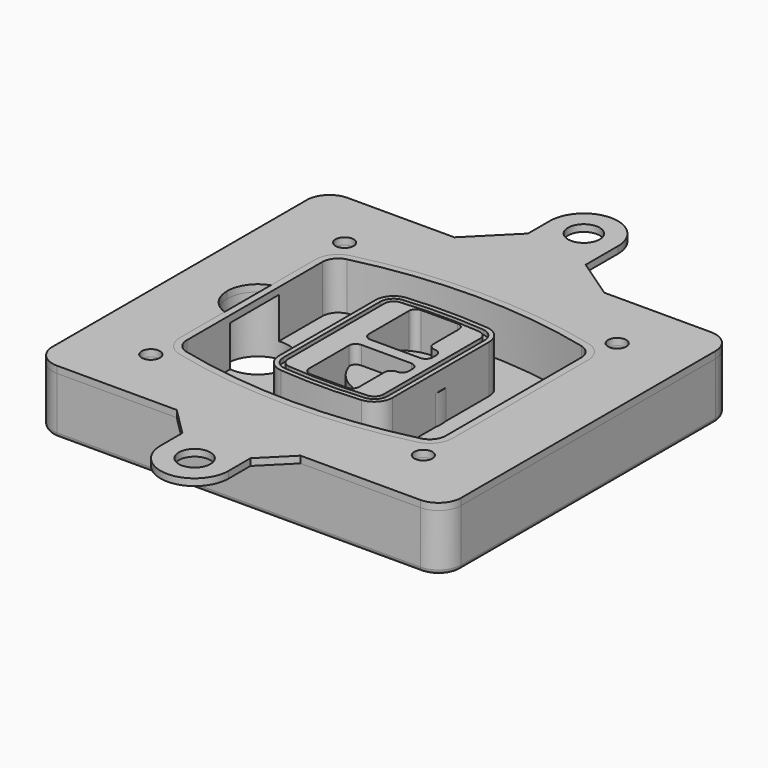
from build123d import *

# Parameters (mm, degrees)
F0_R      = 4
F1_DEPTH  = 25
F2_DEPTH  = 3
F3_DEPTH  = 18
F5_DEPTH  = 21
F6_DEPTH  = 2
F8_DEPTH  = 20
F9_DEPTH  = 16
F10_DEPTH = 25
F7_R      = 6
F7_R_2    = 4
F11_DEPTH = 6
F13_DEPTH = 9
F15_R     = 2
F16_R     = 6.9644805488
F16_R_2   = 4
F17_DEPTH = 3


# Not quite as in the source:
# - a feature of the source that left no trace in its solid (it failed there, or was rolled back) is left out
# - a feature names something its author has since deleted; it is built from what else it names


with BuildPart() as f1:
    # F0 (on Top) → F1 (new body)
    with BuildSketch(Plane.XY):
        with BuildLine():
            ThreePointArc((-90, -70), (-87.0710678119, -77.0710678119), (-80, -80))
            Line((-80, -80), (80, -80))
            ThreePointArc((80, -80), (87.0710678119, -77.0710678119), (90, -70))
            Line((90, -70), (90, 70))
            ThreePointArc((90, 70), (87.0710678119, 77.0710678119), (80, 80))
            Line((80, 80), (-80, 80))
            ThreePointArc((-80, 80), (-87.0710678119, 77.0710678119), (-90, 70))
            Line((-90, 70), (-90, -70))
        make_face()
        with Locations((-60, -53.3333333333)):
            Circle(F0_R, mode=Mode.SUBTRACT)
        with Locations((60, -53.3333333333)):
            Circle(F0_R, mode=Mode.SUBTRACT)
        with Locations((-60, 53.3333333333)):
            Circle(F0_R, mode=Mode.SUBTRACT)
        with BuildLine():
            ThreePointArc((-64, 37.2990447398), (-61.0143011354, 45.9411029726), (-53.3306899286, 50.8970778549))
            ThreePointArc((-53.3306899286, 50.8970778549), (0, 57.3333333333), (53.3306899286, 50.8970778549))
            ThreePointArc((53.3306899286, 50.8970778549), (61.0143011354, 45.9411029726), (64, 37.2990447398))
            Line((64, 37.2990447398), (64, -37.2990447398))
            ThreePointArc((64, -37.2990447398), (61.0143011354, -45.9411029726), (53.3306899286, -50.8970778549))
            ThreePointArc((53.3306899286, -50.8970778549), (0, -57.3333333333), (-53.3306899286, -50.8970778549))
            ThreePointArc((-53.3306899286, -50.8970778549), (-61.0143011354, -45.9411029726), (-64, -37.2990447398))
            Line((-64, -37.2990447398), (-64, 37.2990447398))
        make_face(mode=Mode.SUBTRACT)
        with Locations((60, 53.3333333333)):
            Circle(F0_R, mode=Mode.SUBTRACT)
        with BuildLine():
            ThreePointArc((53.3306899286, 50.8970778549), (0, 57.3333333333), (-53.3306899286, 50.8970778549))
            ThreePointArc((-53.3306899286, 50.8970778549), (-61.0143011354, 45.9411029726), (-64, 37.2990447398))
            Line((-64, 37.2990447398), (-64, -37.2990447398))
            ThreePointArc((-64, -37.2990447398), (-61.0143011354, -45.9411029726), (-53.3306899286, -50.8970778549))
            ThreePointArc((-53.3306899286, -50.8970778549), (0, -57.3333333333), (53.3306899286, -50.8970778549))
            ThreePointArc((53.3306899286, -50.8970778549), (61.0143011354, -45.9411029726), (64, -37.2990447398))
            Line((64, -37.2990447398), (64, 37.2990447398))
            ThreePointArc((64, 37.2990447398), (61.0143011354, 45.9411029726), (53.3306899286, 50.8970778549))
        make_face()
        with BuildLine():
            Line((-60, -37.2990447398), (-60, 37.2990447398))
            ThreePointArc((-60, 37.2990447398), (-57.8673579538, 43.4719434775), (-52.3790642347, 47.0119255363))
            ThreePointArc((-52.3790642347, 47.0119255363), (0, 53.3333333333), (52.3790642347, 47.0119255363))
            ThreePointArc((52.3790642347, 47.0119255363), (57.8673579538, 43.4719434775), (60, 37.2990447398))
            Line((60, 37.2990447398), (60, -37.2990447398))
            ThreePointArc((60, -37.2990447398), (57.8673579538, -43.4719434775), (52.3790642347, -47.0119255363))
            ThreePointArc((52.3790642347, -47.0119255363), (0, -53.3333333333), (-52.3790642347, -47.0119255363))
            ThreePointArc((-52.3790642347, -47.0119255363), (-57.8673579538, -43.4719434775), (-60, -37.2990447398))
        make_face(mode=Mode.SUBTRACT)
        with BuildLine():
            ThreePointArc((-52.3790642347, 47.0119255363), (-57.8673579538, 43.4719434775), (-60, 37.2990447398))
            Line((-60, 37.2990447398), (-60, -37.2990447398))
            ThreePointArc((-60, -37.2990447398), (-57.8673579538, -43.4719434775), (-52.3790642347, -47.0119255363))
            ThreePointArc((-52.3790642347, -47.0119255363), (0, -53.3333333333), (52.3790642347, -47.0119255363))
            ThreePointArc((52.3790642347, -47.0119255363), (57.8673579538, -43.4719434775), (60, -37.2990447398))
            Line((60, -37.2990447398), (60, 37.2990447398))
            ThreePointArc((60, 37.2990447398), (57.8673579538, 43.4719434775), (52.3790642347, 47.0119255363))
            ThreePointArc((52.3790642347, 47.0119255363), (0, 53.3333333333), (-52.3790642347, 47.0119255363))
        make_face()
        with BuildLine():
            ThreePointArc((51.6653449643, 44.0980612973), (55.5071505677, 41.6200738562), (57, 37.2990447398))
            Line((57, 37.2990447398), (57, -37.2990447398))
            ThreePointArc((57, -37.2990447398), (55.5071505677, -41.6200738562), (51.6653449643, -44.0980612973))
            ThreePointArc((51.6653449643, -44.0980612973), (0, -50.3333333333), (-51.6653449643, -44.0980612973))
            ThreePointArc((-51.6653449643, -44.0980612973), (-55.5071505677, -41.6200738562), (-57, -37.2990447398))
            Line((-57, -37.2990447398), (-57, 37.2990447398))
            ThreePointArc((-57, 37.2990447398), (-55.5071505677, 41.6200738562), (-51.6653449643, 44.0980612973))
            ThreePointArc((-51.6653449643, 44.0980612973), (0, 50.3333333333), (51.6653449643, 44.0980612973))
        make_face(mode=Mode.SUBTRACT)
        with BuildLine():
            Line((57, -37.2990447398), (57, 37.2990447398))
            ThreePointArc((57, 37.2990447398), (55.5071505677, 41.6200738562), (51.6653449643, 44.0980612973))
            ThreePointArc((51.6653449643, 44.0980612973), (0, 50.3333333333), (-51.6653449643, 44.0980612973))
            ThreePointArc((-51.6653449643, 44.0980612973), (-55.5071505677, 41.6200738562), (-57, 37.2990447398))
            Line((-57, 37.2990447398), (-57, -37.2990447398))
            ThreePointArc((-57, -37.2990447398), (-55.5071505677, -41.6200738562), (-51.6653449643, -44.0980612973))
            ThreePointArc((-51.6653449643, -44.0980612973), (0, -50.3333333333), (51.6653449643, -44.0980612973))
            ThreePointArc((51.6653449643, -44.0980612973), (55.5071505677, -41.6200738562), (57, -37.2990447398))
        make_face()
    extrude(amount=-F1_DEPTH)

    # F0 (on Top) → F2 (join)
    with BuildSketch(Plane.XY):
        with BuildLine():
            ThreePointArc((-52.3790642347, 47.0119255363), (-57.8673579538, 43.4719434775), (-60, 37.2990447398))
            Line((-60, 37.2990447398), (-60, -37.2990447398))
            ThreePointArc((-60, -37.2990447398), (-57.8673579538, -43.4719434775), (-52.3790642347, -47.0119255363))
            ThreePointArc((-52.3790642347, -47.0119255363), (0, -53.3333333333), (52.3790642347, -47.0119255363))
            ThreePointArc((52.3790642347, -47.0119255363), (57.8673579538, -43.4719434775), (60, -37.2990447398))
            Line((60, -37.2990447398), (60, 37.2990447398))
            ThreePointArc((60, 37.2990447398), (57.8673579538, 43.4719434775), (52.3790642347, 47.0119255363))
            ThreePointArc((52.3790642347, 47.0119255363), (0, 53.3333333333), (-52.3790642347, 47.0119255363))
        make_face()
        with BuildLine():
            ThreePointArc((51.6653449643, 44.0980612973), (55.5071505677, 41.6200738562), (57, 37.2990447398))
            Line((57, 37.2990447398), (57, -37.2990447398))
            ThreePointArc((57, -37.2990447398), (55.5071505677, -41.6200738562), (51.6653449643, -44.0980612973))
            ThreePointArc((51.6653449643, -44.0980612973), (0, -50.3333333333), (-51.6653449643, -44.0980612973))
            ThreePointArc((-51.6653449643, -44.0980612973), (-55.5071505677, -41.6200738562), (-57, -37.2990447398))
            Line((-57, -37.2990447398), (-57, 37.2990447398))
            ThreePointArc((-57, 37.2990447398), (-55.5071505677, 41.6200738562), (-51.6653449643, 44.0980612973))
            ThreePointArc((-51.6653449643, 44.0980612973), (0, 50.3333333333), (51.6653449643, 44.0980612973))
        make_face(mode=Mode.SUBTRACT)
    extrude(amount=F2_DEPTH)

    # F0 (on Top) → F3 (cut)
    with BuildSketch(Plane.XY):
        with BuildLine():
            Line((57, -37.2990447398), (57, 37.2990447398))
            ThreePointArc((57, 37.2990447398), (55.5071505677, 41.6200738562), (51.6653449643, 44.0980612973))
            ThreePointArc((51.6653449643, 44.0980612973), (0, 50.3333333333), (-51.6653449643, 44.0980612973))
            ThreePointArc((-51.6653449643, 44.0980612973), (-55.5071505677, 41.6200738562), (-57, 37.2990447398))
            Line((-57, 37.2990447398), (-57, -37.2990447398))
            ThreePointArc((-57, -37.2990447398), (-55.5071505677, -41.6200738562), (-51.6653449643, -44.0980612973))
            ThreePointArc((-51.6653449643, -44.0980612973), (0, -50.3333333333), (51.6653449643, -44.0980612973))
            ThreePointArc((51.6653449643, -44.0980612973), (55.5071505677, -41.6200738562), (57, -37.2990447398))
        make_face()
    extrude(amount=-F3_DEPTH, mode=Mode.SUBTRACT)

    # F4 (on face) → F5 (join, through all)
    with BuildSketch(Plane.XY.offset(3)):
        with BuildLine():
            ThreePointArc((-25, -26.587695628), (-22.8992979869, -31.9912392117), (-17.7004291845, -34.5569740744))
            ThreePointArc((-17.7004291845, -34.5569740744), (0, -35.3333333333), (17.7004291845, -34.5569740744))
            ThreePointArc((17.7004291845, -34.5569740744), (22.8992979869, -31.9912392117), (25, -26.587695628))
            Line((25, -26.587695628), (25, 26.587695628))
            ThreePointArc((25, 26.587695628), (22.8992979869, 31.9912392117), (17.7004291845, 34.5569740744))
            ThreePointArc((17.7004291845, 34.5569740744), (0, 35.3333333333), (-17.7004291845, 34.5569740744))
            ThreePointArc((-17.7004291845, 34.5569740744), (-22.8992979869, 31.9912392117), (-25, 26.587695628))
            Line((-25, 26.587695628), (-25, -26.587695628))
        make_face()
        with BuildLine():
            ThreePointArc((17.5253218884, 32.5646544628), (21.4244734902, 30.6403533158), (23, 26.587695628))
            Line((23, 26.587695628), (23, -26.587695628))
            ThreePointArc((23, -26.587695628), (21.4244734902, -30.6403533158), (17.5253218884, -32.5646544628))
            ThreePointArc((17.5253218884, -32.5646544628), (0, -33.3333333333), (-17.5253218884, -32.5646544628))
            ThreePointArc((-17.5253218884, -32.5646544628), (-21.4244734902, -30.6403533158), (-23, -26.587695628))
            Line((-23, -26.587695628), (-23, 26.587695628))
            ThreePointArc((-23, 26.587695628), (-21.4244734902, 30.6403533158), (-17.5253218884, 32.5646544628))
            ThreePointArc((-17.5253218884, 32.5646544628), (0, 33.3333333333), (17.5253218884, 32.5646544628))
        make_face(mode=Mode.SUBTRACT)
        with BuildLine():
            Line((23, -26.587695628), (23, 26.587695628))
            ThreePointArc((23, 26.587695628), (21.4244734902, 30.6403533158), (17.5253218884, 32.5646544628))
            ThreePointArc((17.5253218884, 32.5646544628), (0, 33.3333333333), (-17.5253218884, 32.5646544628))
            ThreePointArc((-17.5253218884, 32.5646544628), (-21.4244734902, 30.6403533158), (-23, 26.587695628))
            Line((-23, 26.587695628), (-23, -26.587695628))
            ThreePointArc((-23, -26.587695628), (-21.4244734902, -30.6403533158), (-17.5253218884, -32.5646544628))
            ThreePointArc((-17.5253218884, -32.5646544628), (0, -33.3333333333), (17.5253218884, -32.5646544628))
            ThreePointArc((17.5253218884, -32.5646544628), (21.4244734902, -30.6403533158), (23, -26.587695628))
        make_face()
        with BuildLine():
            ThreePointArc((17.3502145923, 30.5723348512), (19.9496489934, 29.2894674198), (21, 26.587695628))
            Line((21, 26.587695628), (21, -26.587695628))
            ThreePointArc((21, -26.587695628), (19.9496489934, -29.2894674198), (17.3502145923, -30.5723348512))
            ThreePointArc((17.3502145923, -30.5723348512), (0, -31.3333333333), (-17.3502145923, -30.5723348512))
            ThreePointArc((-17.3502145923, -30.5723348512), (-19.9496489934, -29.2894674198), (-21, -26.587695628))
            Line((-21, -26.587695628), (-21, 26.587695628))
            ThreePointArc((-21, 26.587695628), (-19.9496489934, 29.2894674198), (-17.3502145923, 30.5723348512))
            ThreePointArc((-17.3502145923, 30.5723348512), (0, 31.3333333333), (17.3502145923, 30.5723348512))
        make_face(mode=Mode.SUBTRACT)
        with BuildLine():
            Line((21, -26.587695628), (21, 26.587695628))
            ThreePointArc((21, 26.587695628), (19.9496489934, 29.2894674198), (17.3502145923, 30.5723348512))
            ThreePointArc((17.3502145923, 30.5723348512), (0, 31.3333333333), (-17.3502145923, 30.5723348512))
            ThreePointArc((-17.3502145923, 30.5723348512), (-19.9496489934, 29.2894674198), (-21, 26.587695628))
            Line((-21, 26.587695628), (-21, -26.587695628))
            ThreePointArc((-21, -26.587695628), (-19.9496489934, -29.2894674198), (-17.3502145923, -30.5723348512))
            ThreePointArc((-17.3502145923, -30.5723348512), (0, -31.3333333333), (17.3502145923, -30.5723348512))
            ThreePointArc((17.3502145923, -30.5723348512), (19.9496489934, -29.2894674198), (21, -26.587695628))
        make_face()
        with BuildLine():
            Line((-8, -2.5), (14, -2.5))
            ThreePointArc((14, -2.5), (16.1213203436, -3.3786796564), (17, -5.5))
            Line((17, -5.5), (17, -7.5))
            ThreePointArc((17, -7.5), (16.1213203436, -9.6213203436), (14, -10.5))
            ThreePointArc((14, -10.5), (11.8786796564, -11.3786796564), (11, -13.5))
            Line((11, -13.5), (11, -27.5))
            ThreePointArc((11, -27.5), (10.1213203436, -29.6213203436), (8, -30.5))
            Line((8, -30.5), (-8, -30.5))
            ThreePointArc((-8, -30.5), (-10.1213203436, -29.6213203436), (-11, -27.5))
            Line((-11, -27.5), (-11, -5.5))
            ThreePointArc((-11, -5.5), (-10.1213203436, -3.3786796564), (-8, -2.5))
        make_face(mode=Mode.SUBTRACT)
        with BuildLine():
            ThreePointArc((-8, 2.5), (-10.1213203436, 3.3786796564), (-11, 5.5))
            Line((-11, 5.5), (-11, 27.5))
            ThreePointArc((-11, 27.5), (-10.1213203436, 29.6213203436), (-8, 30.5))
            Line((-8, 30.5), (8, 30.5))
            ThreePointArc((8, 30.5), (10.1213203436, 29.6213203436), (11, 27.5))
            Line((11, 27.5), (11, 13.5))
            ThreePointArc((11, 13.5), (11.8786796564, 11.3786796564), (14, 10.5))
            ThreePointArc((14, 10.5), (16.1213203436, 9.6213203436), (17, 7.5))
            Line((17, 7.5), (17, 5.5))
            ThreePointArc((17, 5.5), (16.1213203436, 3.3786796564), (14, 2.5))
            Line((14, 2.5), (-8, 2.5))
        make_face(mode=Mode.SUBTRACT)
    extrude(amount=-F5_DEPTH)

    # F4 (on face) → F6 (cut)
    with BuildSketch(Plane.XY.offset(3)):
        with BuildLine():
            Line((23, -26.587695628), (23, 26.587695628))
            ThreePointArc((23, 26.587695628), (21.4244734902, 30.6403533158), (17.5253218884, 32.5646544628))
            ThreePointArc((17.5253218884, 32.5646544628), (0, 33.3333333333), (-17.5253218884, 32.5646544628))
            ThreePointArc((-17.5253218884, 32.5646544628), (-21.4244734902, 30.6403533158), (-23, 26.587695628))
            Line((-23, 26.587695628), (-23, -26.587695628))
            ThreePointArc((-23, -26.587695628), (-21.4244734902, -30.6403533158), (-17.5253218884, -32.5646544628))
            ThreePointArc((-17.5253218884, -32.5646544628), (0, -33.3333333333), (17.5253218884, -32.5646544628))
            ThreePointArc((17.5253218884, -32.5646544628), (21.4244734902, -30.6403533158), (23, -26.587695628))
        make_face()
        with BuildLine():
            ThreePointArc((17.3502145923, 30.5723348512), (19.9496489934, 29.2894674198), (21, 26.587695628))
            Line((21, 26.587695628), (21, -26.587695628))
            ThreePointArc((21, -26.587695628), (19.9496489934, -29.2894674198), (17.3502145923, -30.5723348512))
            ThreePointArc((17.3502145923, -30.5723348512), (0, -31.3333333333), (-17.3502145923, -30.5723348512))
            ThreePointArc((-17.3502145923, -30.5723348512), (-19.9496489934, -29.2894674198), (-21, -26.587695628))
            Line((-21, -26.587695628), (-21, 26.587695628))
            ThreePointArc((-21, 26.587695628), (-19.9496489934, 29.2894674198), (-17.3502145923, 30.5723348512))
            ThreePointArc((-17.3502145923, 30.5723348512), (0, 31.3333333333), (17.3502145923, 30.5723348512))
        make_face(mode=Mode.SUBTRACT)
    extrude(amount=-F6_DEPTH, mode=Mode.SUBTRACT)

    # F7 (on face) → F8 (join)
    with BuildSketch(Plane(origin=(0, 0, -25), x_dir=(1, 0, 0), z_dir=(0, 0, -1))):
        with BuildLine():
            ThreePointArc((-6.71157564, 0), (6.7567035675, 13.4682792075), (20.224982775, 0))
            Line((20.224982775, 0), (25.224982775, 0))
            ThreePointArc((25.224982775, 0), (6.7567035675, 18.4682792075), (-11.71157564, 0))
            Line((-11.71157564, 0), (-6.71157564, 0))
        make_face()
        with BuildLine():
            Line((-6.71157564, 0), (20.224982775, 0))
            ThreePointArc((20.224982775, 0), (6.7567035675, 13.4682792075), (-6.71157564, 0))
        make_face()
        with BuildLine():
            ThreePointArc((-6.71157564, 0), (6.7567035675, -13.4682792075), (20.224982775, 0))
            Line((20.224982775, 0), (-6.71157564, 0))
        make_face()
        with BuildLine():
            Line((25.224982775, 0), (20.224982775, 0))
            ThreePointArc((20.224982775, 0), (6.7567035675, -13.4682792075), (-6.71157564, 0))
            Line((-6.71157564, 0), (-11.71157564, 0))
            ThreePointArc((-11.71157564, 0), (6.7567035675, -18.4682792075), (25.224982775, 0))
        make_face()
    extrude(amount=-F8_DEPTH)

    # F7 (on face) → F9 (cut)
    with BuildSketch(Plane(origin=(0, 0, -25), x_dir=(1, 0, 0), z_dir=(0, 0, -1))):
        with BuildLine():
            Line((-6.71157564, 0), (20.224982775, 0))
            ThreePointArc((20.224982775, 0), (6.7567035675, 13.4682792075), (-6.71157564, 0))
        make_face()
        with BuildLine():
            ThreePointArc((-6.71157564, 0), (6.7567035675, -13.4682792075), (20.224982775, 0))
            Line((20.224982775, 0), (-6.71157564, 0))
        make_face()
    extrude(amount=-F9_DEPTH, mode=Mode.SUBTRACT)

    # F7 (on face) → F10 (cut)
    with BuildSketch(Plane(origin=(0, 0, -25), x_dir=(1, 0, 0), z_dir=(0, 0, -1))):
        with BuildLine():
            Line((-69.0318229325, 0), (-42.0952645175, 0))
            ThreePointArc((-42.0952645175, 0), (-55.563543725, 13.4682792075), (-69.0318229325, 0))
        make_face()
        with BuildLine():
            ThreePointArc((-69.0318229325, 0), (-55.563543725, -13.4682792075), (-42.0952645175, 0))
            Line((-42.0952645175, 0), (-69.0318229325, 0))
        make_face()
    extrude(amount=-F10_DEPTH, mode=Mode.SUBTRACT)

    # F7 (on face) → F11 (cut)
    with BuildSketch(Plane(origin=(0, 0, -25), x_dir=(1, 0, 0), z_dir=(0, 0, -1))):
        with Locations((60, -53.3333333333)):
            Circle(F7_R)
        with Locations((60, -53.3333333333)):
            Circle(F7_R_2, mode=Mode.SUBTRACT)
        with Locations((-60, -53.3333333333)):
            Circle(F7_R)
        with Locations((-60, -53.3333333333)):
            Circle(F7_R_2, mode=Mode.SUBTRACT)
        with Locations((-60, 53.3333333333)):
            Circle(F7_R)
        with Locations((-60, 53.3333333333)):
            Circle(F7_R_2, mode=Mode.SUBTRACT)
        with Locations((60, 53.3333333333)):
            Circle(F7_R)
        with Locations((60, 53.3333333333)):
            Circle(F7_R_2, mode=Mode.SUBTRACT)
    extrude(amount=-F11_DEPTH, mode=Mode.SUBTRACT)

    # F12 (on face) → F13 (cut, through all)
    with BuildSketch(Plane(origin=(0, 0, -9), x_dir=(1, 0, 0), z_dir=(0, 0, -1))):
        with BuildLine():
            ThreePointArc((20.224982775, 0), (20.1663399806, 1.2554664788), (19.9909222755, 2.5))
            Line((19.9909222755, 2.5), (14, 2.5))
            ThreePointArc((14, 2.5), (16.1213203436, 3.3786796564), (17, 5.5))
            Line((17, 5.5), (17, 7.5))
            ThreePointArc((17, 7.5), (16.1213203436, 9.6213203436), (14, 10.5))
            ThreePointArc((14, 10.5), (12.1627255951, 11.1284134507), (11.0951631559, 12.750384826))
            ThreePointArc((11.0951631559, 12.750384826), (11.0476113807, 12.7664660322), (11, 12.7823698976))
            Line((11, 12.7823698976), (11, -12.7823698976))
            ThreePointArc((11, -12.7823698976), (11.0476113807, -12.7664660322), (11.0951631559, -12.750384826))
            ThreePointArc((11.0951631559, -12.750384826), (12.1627255951, -11.1284134507), (14, -10.5))
            ThreePointArc((14, -10.5), (16.1213203436, -9.6213203436), (17, -7.5))
            Line((17, -7.5), (17, -5.5))
            ThreePointArc((17, -5.5), (16.1213203436, -3.3786796564), (14, -2.5))
            Line((14, -2.5), (19.9909222755, -2.5))
            ThreePointArc((19.9909222755, -2.5), (20.1663399806, -1.2554664788), (20.224982775, 0))
        make_face()
    extrude(amount=F13_DEPTH, mode=Mode.SUBTRACT)

    # F15
    f15_edges = [f1.edges().sort_by_distance(p)[0] for p in [
        (0, -80, -25),
        (-87.071068, -77.071068, -25),
        (-90, 0, -25),
        (-87.071068, 77.071068, -25),
        (87.071068, -77.071068, -25),
        (0, 80, -25),
        (90, 0, -25),
        (87.071068, 77.071068, -25),
    ]]
    fillet(f15_edges, radius=F15_R)


with BuildPart() as f17:
    # F16 (on face) → F17 (new body, through all)
    with BuildSketch(Plane.XY):
        with BuildLine():
            Line((-15, 98), (-33, 80))
            Line((-33, 80), (33, 80))
            Line((33, 80), (15, 92.25))
            Line((15, 92.25), (15, 110))
            ThreePointArc((15, 110), (0, 125), (-15, 110))
            Line((-15, 110), (-15, 98))
        make_face()
        with Locations((0, 110)):
            Circle(F16_R, mode=Mode.SUBTRACT)
        with BuildLine():
            Line((33, 80), (-33, 80))
            Line((-33, 80), (-80, 80))
            ThreePointArc((-80, 80), (-87.0710678119, 77.0710678119), (-90, 70))
            Line((-90, 70), (-90, -70))
            ThreePointArc((-90, -70), (-87.0710678119, -77.0710678119), (-80, -80))
            Line((-80, -80), (-27.25, -80))
            Line((-27.25, -80), (27.25, -80))
            Line((27.25, -80), (80, -80))
            ThreePointArc((80, -80), (87.0710678119, -77.0710678119), (90, -70))
            Line((90, -70), (90, 70))
            ThreePointArc((90, 70), (87.0710678119, 77.0710678119), (80, 80))
            Line((80, 80), (33, 80))
        make_face()
        with Locations((-60, -53.3333333333)):
            Circle(F16_R_2, mode=Mode.SUBTRACT)
        with BuildLine():
            ThreePointArc((-60, 37.2990447398), (-57.8673579538, 43.4719434775), (-52.3790642347, 47.0119255363))
            ThreePointArc((-52.3790642347, 47.0119255363), (0, 53.3333333333), (52.3790642347, 47.0119255363))
            ThreePointArc((52.3790642347, 47.0119255363), (57.8673579538, 43.4719434775), (60, 37.2990447398))
            Line((60, 37.2990447398), (60, -37.2990447398))
            ThreePointArc((60, -37.2990447398), (57.8673579538, -43.4719434775), (52.3790642347, -47.0119255363))
            ThreePointArc((52.3790642347, -47.0119255363), (0, -53.3333333333), (-52.3790642347, -47.0119255363))
            ThreePointArc((-52.3790642347, -47.0119255363), (-57.8673579538, -43.4719434775), (-60, -37.2990447398))
            Line((-60, -37.2990447398), (-60, -12.7166190685))
            ThreePointArc((-60, -12.7166190685), (-66.5441169481, -7.798817635), (-69.0318229325, 0))
            ThreePointArc((-69.0318229325, 0), (-66.5441169481, 7.798817635), (-60, 12.7166190685))
            Line((-60, 12.7166190685), (-60, 37.2990447398))
        make_face(mode=Mode.SUBTRACT)
        with Locations((60, -53.3333333333)):
            Circle(F16_R_2, mode=Mode.SUBTRACT)
        with Locations((-60, 53.3333333333)):
            Circle(F16_R_2, mode=Mode.SUBTRACT)
        with Locations((60, 53.3333333333)):
            Circle(F16_R_2, mode=Mode.SUBTRACT)
        with BuildLine():
            Line((27.25, -80), (-27.25, -80))
            Line((-27.25, -80), (-15, -92.25))
            Line((-15, -92.25), (-15, -104.25))
            ThreePointArc((-15, -104.25), (0, -119.25), (15, -104.25))
            Line((15, -104.25), (15, -92.25))
            Line((15, -92.25), (27.25, -80))
        make_face()
        with Locations((0, -104.25)):
            Circle(F16_R, mode=Mode.SUBTRACT)
    extrude(amount=F17_DEPTH)


solid = Compound([f1.part, f17.part])
